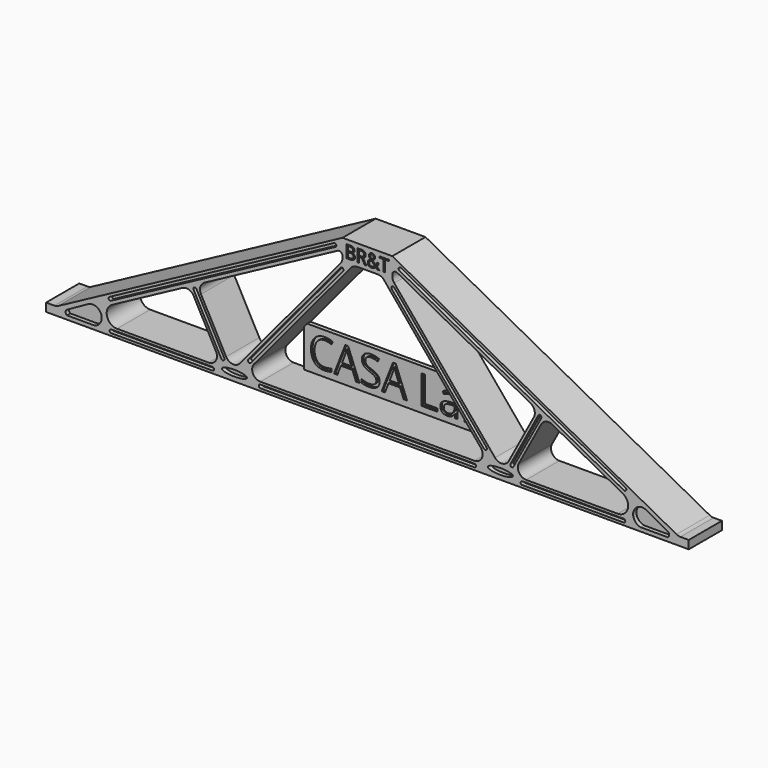
from build123d import *

# Parameters (mm, degrees)
F1_DEPTH     = 25.4
F2_TEXT_SIZE = 10.7261711955
F3_DEPTH     = 1.27
F4_W         = 57.15
F4_H         = 25.4
F5_DEPTH     = 2.54
F6_TEXT_SIZE = 24.6944444444
F7_DEPTH     = 1.27
F9_DEPTH     = 2.54


# Not quite as in the source:
# - Text() gives the source's letters only with a copy of the font that has no kerning and outlines rounded to 1/6400 em; it was checked with that copy


with BuildPart() as f1:
    # F0 (on Front) → F1 (new body)
    with BuildSketch(Plane.XZ):
        with BuildLine():
            Line((0, 99.06), (-15.24, 99.06))
            Line((-15.24, 99.06), (-189.3753994274, 5.6830466838))
            ThreePointArc((-189.3753994274, 5.6830466838), (-190.5384502728, 5.2330677473), (-191.776084539, 5.08))
            Line((-191.776084539, 5.08), (-196.85, 5.08))
            Line((-196.85, 5.08), (-196.85, 0))
            Line((-196.85, 0), (0, 0))
            Line((0, 0), (0, 5.08))
            Line((0, 5.08), (-65.5285182316, 5.08))
            ThreePointArc((-65.5285182316, 5.08), (-70.129039044, 8.0055608027), (-69.4307002655, 13.4125951753))
            Line((-69.4307002655, 13.4125951753), (-10.1498756257, 84.5325951753))
            ThreePointArc((-10.1498756257, 84.5325951753), (-8.4021327891, 85.8805208124), (-6.2476935918, 86.36))
            Line((-6.2476935918, 86.36), (0, 86.36))
            Line((0, 86.36), (0, 99.06))
        make_face()
        with BuildLine():
            ThreePointArc((-92.765172962, 12.5606851116), (-92.8831194896, 7.5512723759), (-97.2421262782, 5.08))
            Line((-97.2421262782, 5.08), (-153.3792186506, 5.08))
            ThreePointArc((-153.3792186506, 5.08), (-159.5378839665, 9.8829571672), (-156.38007504, 17.0261916452))
            Line((-156.38007504, 17.0261916452), (-113.3088863312, 40.1223363151))
            ThreePointArc((-113.3088863312, 40.1223363151), (-109.4400578926, 40.5086077698), (-106.4312479035, 38.0460681105))
            Line((-106.4312479035, 38.0460681105), (-92.765172962, 12.5606851116))
        make_face(mode=Mode.SUBTRACT)
        with BuildLine():
            ThreePointArc((-18.3543770699, 91.0399717161), (-16.2688461426, 90.9908679301), (-15.24, 89.1761155929))
            Line((-15.24, 89.1761155929), (-15.24, 88.1995511723))
            ThreePointArc((-15.24, 88.1995511723), (-15.5435219705, 86.4699102749), (-16.4178179661, 84.946955997))
            Line((-16.4178179661, 84.946955997), (-78.1686074569, 10.8637060545))
            ThreePointArc((-78.1686074569, 10.8637060545), (-82.5846262313, 9.0623550682), (-86.547742807, 11.7156161182))
            Line((-86.547742807, 11.7156161182), (-101.9542945874, 40.4467532221))
            ThreePointArc((-101.9542945874, 40.4467532221), (-102.340566042, 44.3155816607), (-99.8780263828, 47.3243916498))
            Line((-99.8780263828, 47.3243916498), (-18.3543770699, 91.0399717161))
        make_face(mode=Mode.SUBTRACT)
        with BuildLine():
            Line((15.24, 99.06), (0, 99.06))
            Line((0, 99.06), (0, 86.36))
            Line((0, 86.36), (6.2476935918, 86.36))
            ThreePointArc((6.2476935918, 86.36), (8.4021327891, 85.8805208124), (10.1498756257, 84.5325951753))
            Line((10.1498756257, 84.5325951753), (69.4307002655, 13.4125951753))
            ThreePointArc((69.4307002655, 13.4125951753), (70.129039044, 8.0055608027), (65.5285182316, 5.08))
            Line((65.5285182316, 5.08), (0, 5.08))
            Line((0, 5.08), (0, 0))
            Line((0, 0), (196.85, 0))
            Line((196.85, 0), (196.85, 5.08))
            Line((196.85, 5.08), (191.776084539, 5.08))
            ThreePointArc((191.776084539, 5.08), (190.5384502728, 5.2330677473), (189.3753994274, 5.6830466838))
            Line((189.3753994274, 5.6830466838), (15.24, 99.06))
        make_face()
        with BuildLine():
            Line((92.765172962, 12.5606851116), (106.4312479035, 38.0460681105))
            ThreePointArc((106.4312479035, 38.0460681105), (109.4400578926, 40.5086077698), (113.3088863312, 40.1223363151))
            Line((113.3088863312, 40.1223363151), (156.38007504, 17.0261916452))
            ThreePointArc((156.38007504, 17.0261916452), (159.5378839665, 9.8829571672), (153.3792186506, 5.08))
            Line((153.3792186506, 5.08), (97.2421262782, 5.08))
            ThreePointArc((97.2421262782, 5.08), (92.8831194896, 7.5512723759), (92.765172962, 12.5606851116))
        make_face(mode=Mode.SUBTRACT)
        with BuildLine():
            Line((15.24, 88.1995511723), (15.24, 89.1761155929))
            ThreePointArc((15.24, 89.1761155929), (16.2688461426, 90.9908679301), (18.3543770699, 91.0399717161))
            Line((18.3543770699, 91.0399717161), (99.8780263828, 47.3243916498))
            ThreePointArc((99.8780263828, 47.3243916498), (102.340566042, 44.3155816607), (101.9542945874, 40.4467532221))
            Line((101.9542945874, 40.4467532221), (86.547742807, 11.7156161182))
            ThreePointArc((86.547742807, 11.7156161182), (82.5846262313, 9.0623550682), (78.1686074569, 10.8637060545))
            Line((78.1686074569, 10.8637060545), (16.4178179661, 84.946955997))
            ThreePointArc((16.4178179661, 84.946955997), (15.5435219705, 86.4699102749), (15.24, 88.1995511723))
        make_face(mode=Mode.SUBTRACT)
    extrude(amount=F1_DEPTH)

    # F2 (on face) → F3 (cut)
    with BuildSketch(Plane.XZ.offset(25.4)):
        with Locations((-13.97, 88.7971567392)):
            Text('BR&T', F2_TEXT_SIZE, font='Open Sans', text_align=(TextAlign.LEFT, TextAlign.BOTTOM))
    extrude(amount=-F3_DEPTH, mode=Mode.SUBTRACT)

    # F4 (on Front) → F5 (join)
    with BuildSketch(Plane.XZ):
        with Locations((-28.575, 17.78)):
            Rectangle(F4_W, F4_H)
        with Locations((28.575, 17.78)):
            Rectangle(F4_W, F4_H)
    extrude(amount=F5_DEPTH)

    # F6 (on face) → F7 (cut)
    with BuildSketch(Plane.XZ.offset(2.54)):
        with Locations((-54.3586458333, 8.89)):
            Text('CASA Lab', F6_TEXT_SIZE, font='Open Sans', text_align=(TextAlign.LEFT, TextAlign.BOTTOM))
    extrude(amount=-F7_DEPTH, mode=Mode.SUBTRACT)

    # F8 (on face) → F9 (cut)
    with BuildSketch(Plane.XZ.offset(25.4)):
        with BuildLine():
            add(Edge.make_bspline(
                [(-73.7982168794, 4.4845882803), (-73.7982168794, 7.7134934772), (-85.3182934225, 6.0990408788), (-96.8383699656, 4.4845882803), (-85.3182934225, 2.8701356819), (-73.7982168794, 1.2556830834), (-73.7982168794, 4.4845882803)],
                knots=[0, 0, 0, 2.0943951024, 2.0943951024, 4.1887902048, 4.1887902048, 6.2831853072, 6.2831853072, 6.2831853072], degree=2, weights=[1, 0.5, 1, 0.5, 1, 0.5, 1]))
        make_face()
        Polygon((-158.0601017891, 20.7460245713), (-157.0998277444, 18.9552432449), (-19.4561315128, 92.7641818038), (-20.5578661597, 94.479107445), align=None)
        with BuildLine():
            ThreePointArc((-158.0601017891, 20.7460245713), (-158.47535543, 19.3704968858), (-157.0998277444, 18.9552432449))
            Line((-157.0998277444, 18.9552432449), (-158.0601017891, 20.7460245713))
        make_face()
        with BuildLine():
            Line((-20.5578661597, 94.479107445), (-19.4561315128, 92.7641818038))
            ThreePointArc((-19.4561315128, 92.7641818038), (-19.2145991213, 94.1307128891), (-20.5578661597, 94.479107445))
        make_face()
        Polygon((-87.67611417, 10.5949968119), (-104.7163999669, 42.3728270818), (-106.5071812934, 41.4125530372), (-89.4353386236, 9.5758734638), align=None)
        with BuildLine():
            Line((-106.5071812934, 41.4125530372), (-104.7163999669, 42.3728270818))
            ThreePointArc((-104.7163999669, 42.3728270818), (-106.0919276525, 42.7880807227), (-106.5071812934, 41.4125530372))
        make_face()
        with BuildLine():
            ThreePointArc((-89.4353386236, 9.5758734638), (-88.0291442504, 9.1764419422), (-87.67611417, 10.5949968119))
            Line((-87.67611417, 10.5949968119), (-89.4353386236, 9.5758734638))
        make_face()
        Polygon((-16.4178179661, 82.5667274156), (-72.9845529759, 14.702857128), (-71.4146979193, 13.4125951753), (-14.8569451525, 81.2656893455), align=None)
        with BuildLine():
            Line((-71.4146979193, 13.4125951753), (-72.9845529759, 14.702857128))
            ThreePointArc((-72.9845529759, 14.702857128), (-72.8403178757, 13.2781989822), (-71.4146979193, 13.4125951753))
        make_face()
        with BuildLine():
            ThreePointArc((-14.8569451525, 81.2656893455), (-14.9868625242, 82.6966447873), (-16.4178179661, 82.5667274156))
            Line((-16.4178179661, 82.5667274156), (-14.8569451525, 81.2656893455))
        make_face()
        Polygon((-94.8418527842, 3.556), (-156.8137705326, 3.556), (-156.9442451, 1.524), (-94.8418527842, 1.524), align=None)
        with BuildLine():
            Line((-156.9442451, 1.524), (-156.8137705326, 3.556))
            ThreePointArc((-156.8137705326, 3.556), (-157.9623373862, 2.6095605103), (-156.9442451, 1.524))
        make_face()
        with BuildLine():
            ThreePointArc((-94.8418527842, 1.524), (-93.8258527842, 2.54), (-94.8418527842, 3.556))
            Line((-94.8418527842, 3.556), (-94.8418527842, 1.524))
        make_face()
        with BuildLine():
            Line((-171.0083186626, 12.6641159877), (-183.9635521173, 5.4495236836))
            ThreePointArc((-183.9635521173, 5.4495236836), (-184.8883027746, 3.9201475588), (-184.0411275625, 2.346473746))
            Line((-184.0411275625, 2.346473746), (-167.5173938274, 2.346473746))
            ThreePointArc((-167.5173938274, 2.346473746), (-163.0688672611, 9.6010013729), (-171.0083186626, 12.6641159877))
        make_face()
        Polygon((65.5285182316, 3.556), (0, 3.556), (-65.5285182316, 3.556), (-65.5285182316, 1.524), (0, 1.524), (65.5285182316, 1.524), align=None)
        with BuildLine():
            Line((-65.5285182316, 1.524), (-65.5285182316, 3.556))
            ThreePointArc((-65.5285182316, 3.556), (-66.5445182316, 2.54), (-65.5285182316, 1.524))
        make_face()
        with BuildLine():
            ThreePointArc((65.5285182316, 1.524), (66.5445182316, 2.54), (65.5285182316, 3.556))
            Line((65.5285182316, 3.556), (65.5285182316, 1.524))
        make_face()
        with BuildLine():
            ThreePointArc((71.4146979193, 13.4125951753), (72.8403178757, 13.2781989822), (72.9845529759, 14.702857128))
            Line((72.9845529759, 14.702857128), (71.4146979193, 13.4125951753))
        make_face()
        Polygon((71.4146979193, 13.4125951753), (72.9845529759, 14.702857128), (16.4178179661, 82.5667274156), (14.8569451525, 81.2656893455), align=None)
        with BuildLine():
            Line((14.8569451525, 81.2656893455), (16.4178179661, 82.5667274156))
            ThreePointArc((16.4178179661, 82.5667274156), (14.9868625242, 82.6966447873), (14.8569451525, 81.2656893455))
        make_face()
        Polygon((19.4561315128, 92.7641818038), (157.0998277444, 18.9552432449), (158.0601017891, 20.7460245713), (20.5578661597, 94.479107445), align=None)
        with BuildLine():
            Line((158.0601017891, 20.7460245713), (157.0998277444, 18.9552432449))
            ThreePointArc((157.0998277444, 18.9552432449), (158.47535543, 19.3704968858), (158.0601017891, 20.7460245713))
        make_face()
        with BuildLine():
            ThreePointArc((20.5578661597, 94.479107445), (19.2145991213, 94.1307128891), (19.4561315128, 92.7641818038))
            Line((19.4561315128, 92.7641818038), (20.5578661597, 94.479107445))
        make_face()
        Polygon((94.8418527842, 1.524), (156.9442451, 1.524), (156.8137705326, 3.556), (94.8418527842, 3.556), align=None)
        with BuildLine():
            Line((156.8137705326, 3.556), (156.9442451, 1.524))
            ThreePointArc((156.9442451, 1.524), (157.9623373862, 2.6095605103), (156.8137705326, 3.556))
        make_face()
        with BuildLine():
            ThreePointArc((94.8418527842, 3.556), (93.8258527842, 2.54), (94.8418527842, 1.524))
            Line((94.8418527842, 1.524), (94.8418527842, 3.556))
        make_face()
        with BuildLine():
            ThreePointArc((106.5071812934, 41.4125530372), (106.0919276525, 42.7880807227), (104.7163999669, 42.3728270818))
            Line((104.7163999669, 42.3728270818), (106.5071812934, 41.4125530372))
        make_face()
        Polygon((106.5071812934, 41.4125530372), (104.7163999669, 42.3728270818), (87.67611417, 10.5949968119), (89.4353386236, 9.5758734638), align=None)
        with BuildLine():
            Line((89.4353386236, 9.5758734638), (87.67611417, 10.5949968119))
            ThreePointArc((87.67611417, 10.5949968119), (88.0291442504, 9.1764419422), (89.4353386236, 9.5758734638))
        make_face()
        with BuildLine():
            ThreePointArc((184.0411275625, 2.346473746), (184.8883027746, 3.9201475588), (183.9635521173, 5.4495236836))
            Line((183.9635521173, 5.4495236836), (171.0083186626, 12.6641159877))
            ThreePointArc((171.0083186626, 12.6641159877), (163.0688672611, 9.6010013729), (167.5173938274, 2.346473746))
            Line((167.5173938274, 2.346473746), (184.0411275625, 2.346473746))
        make_face()
        with BuildLine():
            add(Edge.make_bspline(
                [(73.7982168794, 4.4845882803), (73.7982168794, 1.2556830834), (85.3182934225, 2.8701356819), (96.8383699656, 4.4845882803), (85.3182934225, 6.0990408788), (73.7982168794, 7.7134934772), (73.7982168794, 4.4845882803)],
                knots=[0, 0, 0, 2.0943951024, 2.0943951024, 4.1887902048, 4.1887902048, 6.2831853072, 6.2831853072, 6.2831853072], degree=2, weights=[1, 0.5, 1, 0.5, 1, 0.5, 1]))
        make_face()
    extrude(amount=-F9_DEPTH, mode=Mode.SUBTRACT)


solid = f1.part
